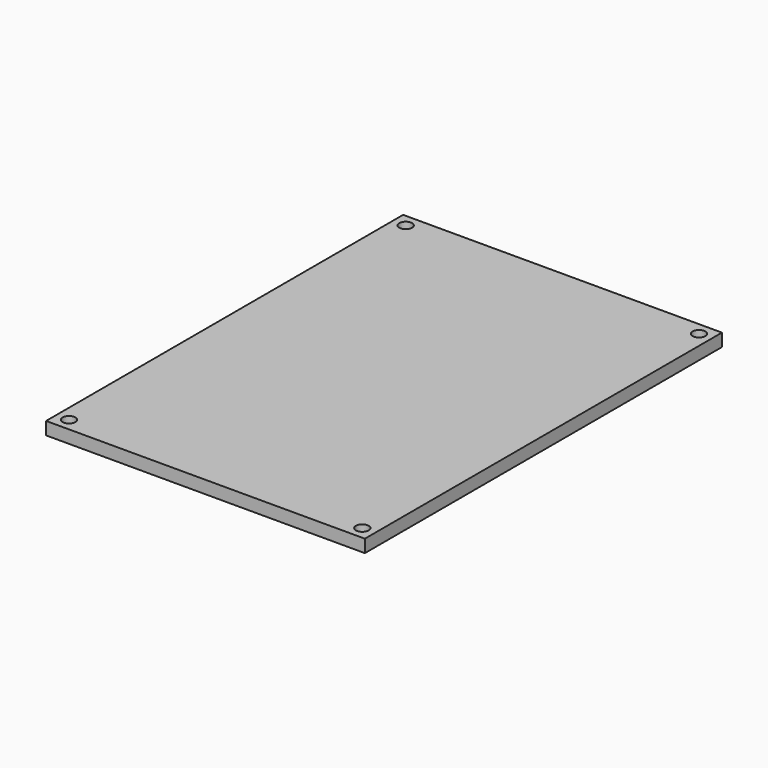
from build123d import *

# Parameters (mm, degrees)
F3_W     = 50
F3_H     = 70
F3_R     = 1
F4_DEPTH = 2


# Not quite as in the source:
# - the program builds the solid bodies; features that only make, move or delete a surface that nothing else refers to are left out


with BuildPart() as f4:
    # F3 (on Top) → F4 (new body)
    with BuildSketch(Plane.XY):
        with Locations((-25, -35)):
            Rectangle(F3_W, F3_H)
        with Locations((-48, -68)):
            Circle(F3_R, mode=Mode.SUBTRACT)
        with Locations((-2, -68)):
            Circle(F3_R, mode=Mode.SUBTRACT)
        with Locations((-48, -2)):
            Circle(F3_R, mode=Mode.SUBTRACT)
        with Locations((-2, -2)):
            Circle(F3_R, mode=Mode.SUBTRACT)
    extrude(amount=F4_DEPTH)


solid = f4.part
